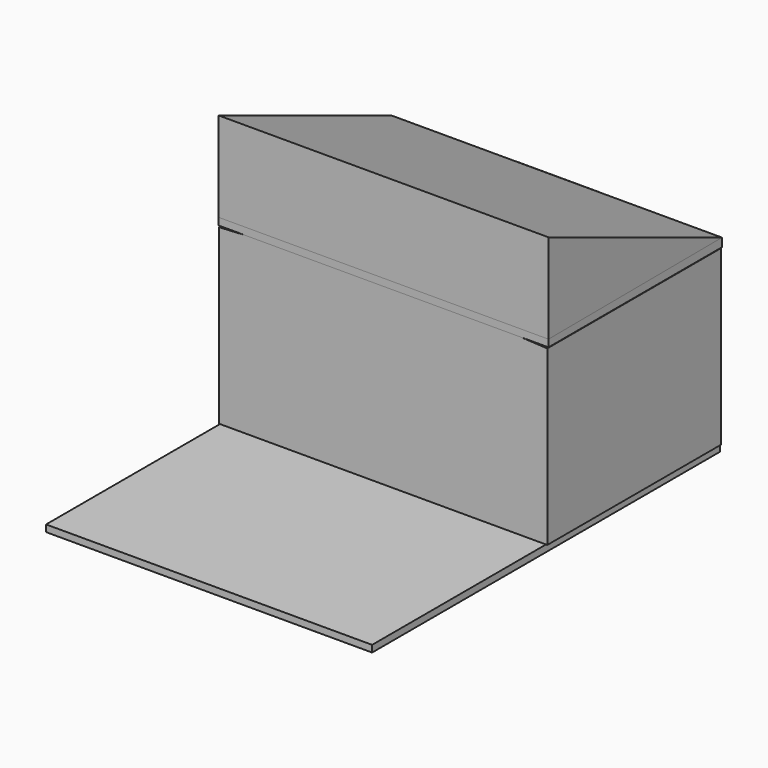
from build123d import *

# Parameters (mm, degrees)
F2_DEPTH  = 2438.4
F4_DEPTH  = 1856.74
F5_DEPTH  = 1844.04
F8_DEPTH  = 3700.78
F9_W      = 936.4943000793
F9_H      = 90.7669610977
F10_DEPTH = 25.4
F0_W      = 3657.6
F0_H      = 4876.8
F11_DEPTH = 76.2


with BuildPart() as f2:
    # F1 (on Front) → F2 (new body)
    with BuildSketch(Plane.XZ):
        Polygon((-1839.4869565964, 0), (1843.4273004532, 0), (1843.4273004532, 1941.2330389023), (0, 2036.8278026581), (-1839.4869565964, 1941.2330389023), align=None)
    extrude(amount=-F2_DEPTH)

    # F9 (on face) → F10 (join)
    with BuildSketch(Plane(origin=(0, 2438.4, 0), x_dir=(-1, 0, 0), z_dir=(0, 1, 0))):
        Polygon((-457.2, 0), (0, 0), (479.2943000793, 0), (479.2943000793, 1941.2330389023), (-457.2, 1941.2330389023), align=None)
        with Locations((11.0471500397, 1986.6165194511)):
            Rectangle(F9_W, F9_H)
    extrude(amount=F10_DEPTH)

    # F0 (on Top) → F11 (join)
    with BuildSketch(Plane.XY):
        Rectangle(F0_W, F0_H)
    extrude(amount=-F11_DEPTH)


with BuildPart() as f4:
    # F3 (on Right) → F4 (new body)
    with BuildSketch(Plane.YZ):
        Polygon((0, 2036.8278026581), (2432.2454929352, 2051.9218444824), (0, 3043.0884361267), align=None)
    extrude(amount=F4_DEPTH)

    # F5 (add): a face of the model
    f5_faces = [f4.faces().sort_by_distance(p)[0] for p in [
        (0, 810.7484976451, 2377.2793610891),
    ]]
    extrude(f5_faces, amount=F5_DEPTH)


with BuildPart() as f8:
    # F6 (on face) → F8 (new body)
    with BuildSketch(Plane(origin=(-1844.04, 0, 0), x_dir=(0, -1, 0), z_dir=(-1, 0, 0))):
        Polygon((0, 2036.8278026581), (-2432.2454929352, 2051.9218444824), (-2432.2454929352, 1956.1679363251), (0, 1956.1679363251), align=None)
    extrude(amount=-F8_DEPTH)


solid = Compound([f2.part, f4.part, f8.part])
